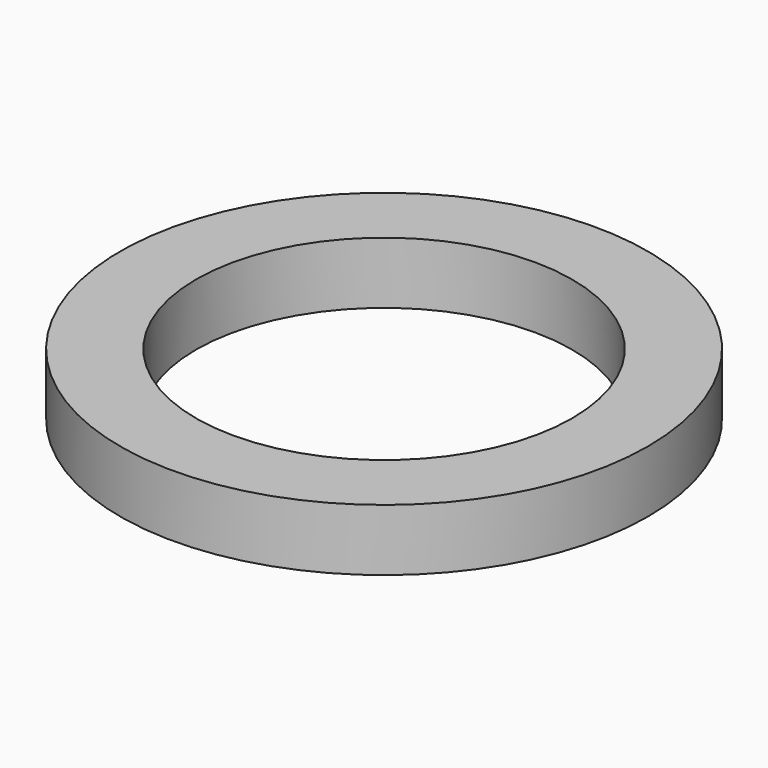
from build123d import *

# Parameters (mm, degrees)
F0_R     = 10.847122292
F0_R_2   = 7.7277782914
F1_DEPTH = 94.742
F3_T     = -2.54


# Not quite as in the source:
# - a feature names something its author has since deleted; it is built from what else it names


with BuildPart() as f1:
    # F0 (on Top) → F1 (new body)
    with BuildSketch(Plane.XY):
        Circle(F0_R)
        Circle(F0_R_2, mode=Mode.SUBTRACT)
    extrude(amount=-F1_DEPTH)

    # F3
    f3_openings = [f1.faces().sort_by_distance(p)[0] for p in [
        (-10.847122, 0, -47.371),
        (-10.540319, 0, 0),
        (-7.727778, 0, -47.371),
    ]]
    offset(amount=F3_T, openings=f3_openings)


solid = f1.part
